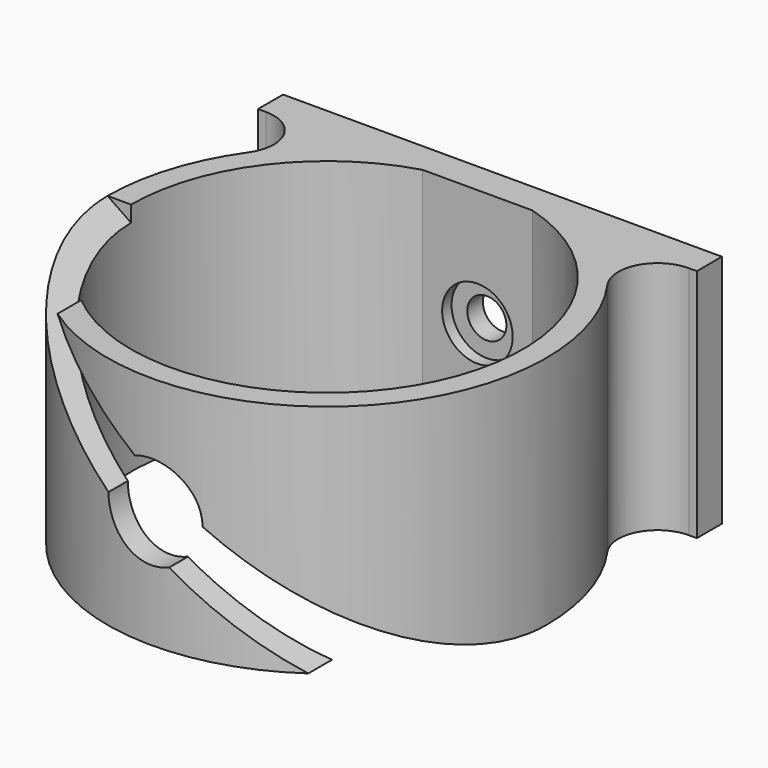
from build123d import *

# Parameters (mm, degrees)
F1_DEPTH       = 30
F2_R           = 5
F4_START       = -28
F4_DEPTH       = 28.001
F6_D           = 5
F6_CBORE_D     = 9
F6_CBORE_DEPTH = 1.5
F7_D           = 12
F7_DEPTH       = 52.001


with BuildPart() as f1:
    # F0 (on Top) → F1 (new body)
    with BuildSketch(Plane.XY):
        with BuildLine():
            ThreePointArc((7, 24), (0, -25), (-7, 24))
            Line((-7, 24), (-14.4222051019, 24))
            ThreePointArc((-14.4222051019, 24), (0, -28), (14.4222051019, 24))
            Line((14.4222051019, 24), (7, 24))
        make_face()
        Polygon((-14.4222051019, 24), (-7, 24), (7, 24), (14.4222051019, 24), (28, 24), (28, 28), (-28, 28), (-28, 24), align=None)
    extrude(amount=F1_DEPTH)

    # F2
    f2_edges = [f1.edges().sort_by_distance(p)[0] for p in [
        (-14.422205, 24, 15),
        (14.422205, 24, 15),
    ]]
    fillet(f2_edges, radius=F2_R)

    # F3 (on face) → F4 (cut)
    with BuildSketch(Plane(origin=(0, 28, 0), x_dir=(-1, 0, 0), z_dir=(0, 1, 0)).offset(F4_START)):
        Polygon((28, 30), (16, 30), (-28, 0), (-16, 0), align=None)
    extrude(amount=-F4_DEPTH, mode=Mode.SUBTRACT)

    # F6 (through all)
    with Locations(Plane.XZ.offset(-24)):
        with Locations((0, 15)):
            CounterBoreHole(F6_D / 2, F6_CBORE_D / 2, F6_CBORE_DEPTH)

    # F7 (through all, one way)
    with BuildSketch(Plane(origin=(0, 24, 0), x_dir=(1, 0, 0), z_dir=(0, 1, 0))):
        with Locations((0, -15)):
            Circle(F7_D / 2)
    extrude(amount=-F7_DEPTH, mode=Mode.SUBTRACT)


solid = f1.part
